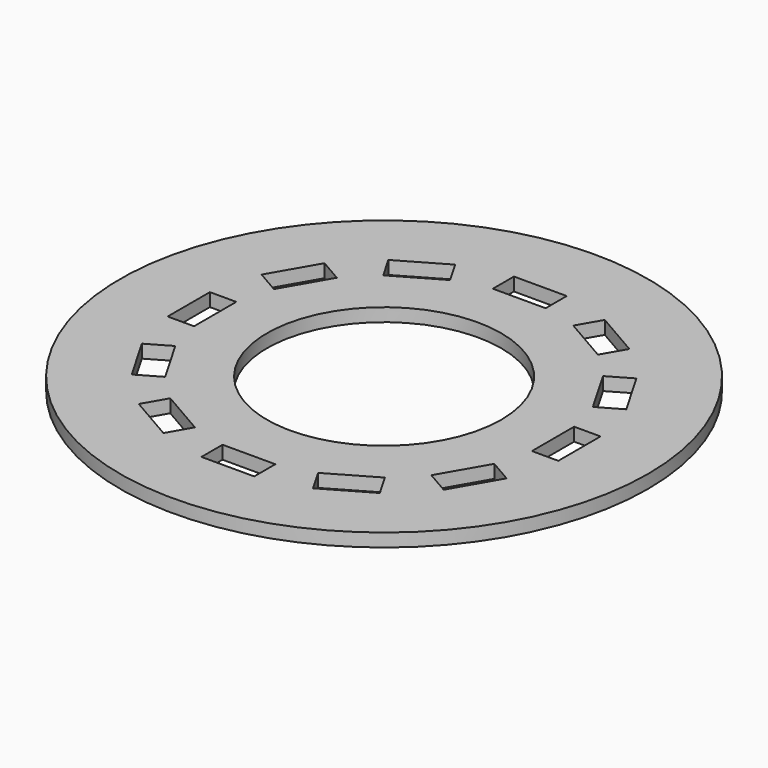
from build123d import *

# Parameters (mm, degrees)
F0_R            = 63.5
F0_R_2          = 28.194
F1_DEPTH        = 3.175
F2_W            = 12.7
F2_H            = 6.35
F3_DEPTH        = 3.176
F3_COPIES_COUNT = 12


# Not quite as in the source:
# - a pattern or mirror of a feature is missing from the dataset's text; its kind, count and spacing are read off the source's solid


with BuildPart() as f1:
    # F0 (on Top) → F1 (new body)
    with BuildSketch(Plane.XY):
        Circle(F0_R)
        Circle(F0_R_2, mode=Mode.SUBTRACT)
    extrude(amount=F1_DEPTH)

    # F2 (on face) → F3 (cut, through all)
    with BuildSketch(Plane.XY.offset(3.175)):
        with Locations((0, 43.815)):
            Rectangle(F2_W, F2_H)
    f3 = extrude(amount=-F3_DEPTH, mode=Mode.SUBTRACT)

    # F3_copies: F3 ×12 about axis
    f3_copies_axis = Axis((0, 0, 0), (0, 0, 1))
    for i in range(1, F3_COPIES_COUNT):
        add(f3.rotate(f3_copies_axis, i * 360 / F3_COPIES_COUNT), mode=Mode.SUBTRACT)


solid = f1.part
